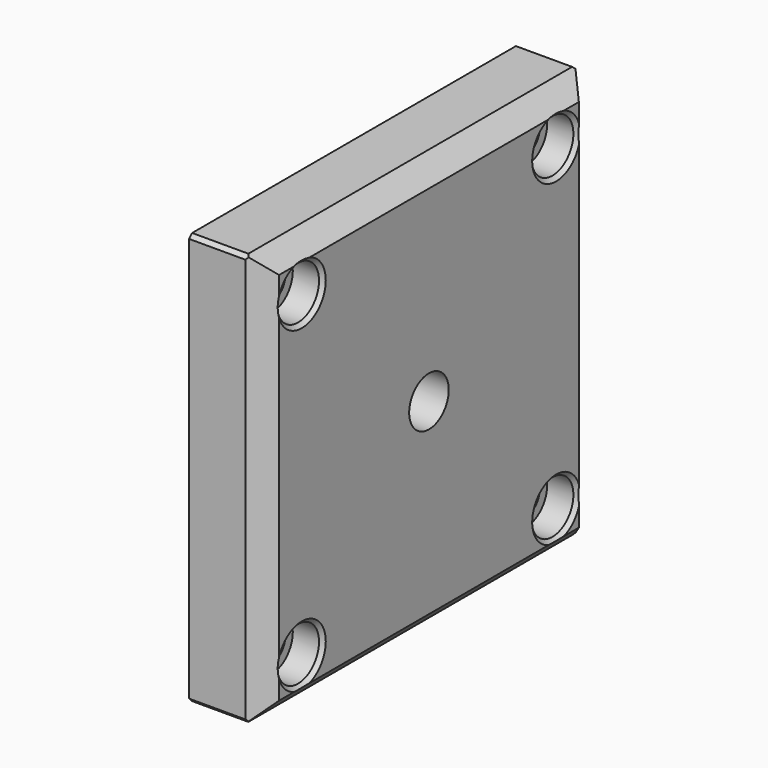
from build123d import *

# Parameters (mm, degrees)
F0_W        = 110
F0_H        = 110
F0_R        = 7
F0_R_2      = 6.6
F0_R_3      = 4.5
F0_R_4      = 5.5
F1_DEPTH    = 20
F2_DEPTH    = 20.001
F3_DEPTH    = 8
F4_DEPTH    = 9.4
F5_SIZE     = 1
F6_T1_DEPTH = 133.7168298797
F6_T3_DEPTH = 133.7168298797
F7_SIZE     = 0.5


# Not quite as in the source:
# - a fillet or chamfer that OpenCascade refuses, or shapes differently, is made with other operations: its cross-section is extruded or revolved along the edge and cut away or added


with BuildPart() as f1:
    # F0 (on Right) → F1 (new body)
    with BuildSketch(Plane.YZ):
        Rectangle(F0_W, F0_H)
        with Locations((-42.4264068712, -42.4264068712)):
            Circle(F0_R, mode=Mode.SUBTRACT)
        with Locations((42.4264068712, -42.4264068712)):
            Circle(F0_R, mode=Mode.SUBTRACT)
        with Locations((-42.4264068712, 42.4264068712)):
            Circle(F0_R, mode=Mode.SUBTRACT)
        Circle(F0_R_2, mode=Mode.SUBTRACT)
        with Locations((42.4264068712, 42.4264068712)):
            Circle(F0_R, mode=Mode.SUBTRACT)
        with Locations((-42.4264068712, 42.4264068712)):
            Circle(F0_R)
        with Locations((-42.4264068712, 42.4264068712)):
            Circle(F0_R_3, mode=Mode.SUBTRACT)
        with Locations((-42.4264068712, -42.4264068712)):
            Circle(F0_R)
        with Locations((-42.4264068712, -42.4264068712)):
            Circle(F0_R_3, mode=Mode.SUBTRACT)
        with Locations((42.4264068712, -42.4264068712)):
            Circle(F0_R)
        with Locations((42.4264068712, -42.4264068712)):
            Circle(F0_R_3, mode=Mode.SUBTRACT)
        with Locations((42.4264068712, 42.4264068712)):
            Circle(F0_R)
        with Locations((42.4264068712, 42.4264068712)):
            Circle(F0_R_3, mode=Mode.SUBTRACT)
        Circle(F0_R_2)
        Circle(F0_R_4, mode=Mode.SUBTRACT)
        Circle(F0_R_4)
        with Locations((-42.4264068712, 42.4264068712)):
            Circle(F0_R_3)
        with Locations((-42.4264068712, -42.4264068712)):
            Circle(F0_R_3)
        with Locations((42.4264068712, -42.4264068712)):
            Circle(F0_R_3)
        with Locations((42.4264068712, 42.4264068712)):
            Circle(F0_R_3)
    extrude(amount=-F1_DEPTH)

    # F0 (on Right) → F2 (cut, through all)
    with BuildSketch(Plane.YZ):
        with Locations((-42.4264068712, 42.4264068712)):
            Circle(F0_R_3)
        with Locations((42.4264068712, -42.4264068712)):
            Circle(F0_R_3)
        with Locations((-42.4264068712, -42.4264068712)):
            Circle(F0_R_3)
        Circle(F0_R_4)
        with Locations((42.4264068712, 42.4264068712)):
            Circle(F0_R_3)
    extrude(amount=-F2_DEPTH, mode=Mode.SUBTRACT)

    # F0 (on Right) → F3 (cut)
    with BuildSketch(Plane.YZ):
        with Locations((-42.4264068712, 42.4264068712)):
            Circle(F0_R)
        with Locations((-42.4264068712, 42.4264068712)):
            Circle(F0_R_3, mode=Mode.SUBTRACT)
        with Locations((42.4264068712, 42.4264068712)):
            Circle(F0_R)
        with Locations((42.4264068712, 42.4264068712)):
            Circle(F0_R_3, mode=Mode.SUBTRACT)
        with Locations((-42.4264068712, -42.4264068712)):
            Circle(F0_R)
        with Locations((-42.4264068712, -42.4264068712)):
            Circle(F0_R_3, mode=Mode.SUBTRACT)
        with Locations((42.4264068712, -42.4264068712)):
            Circle(F0_R)
        with Locations((42.4264068712, -42.4264068712)):
            Circle(F0_R_3, mode=Mode.SUBTRACT)
    extrude(amount=-F3_DEPTH, mode=Mode.SUBTRACT)

    # F0 (on Right) → F4 (cut)
    with BuildSketch(Plane.YZ):
        Circle(F0_R_2)
        Circle(F0_R_4, mode=Mode.SUBTRACT)
    extrude(amount=-F4_DEPTH, mode=Mode.SUBTRACT)

    # F5
    f5_edges = [f1.edges().sort_by_distance(p)[0] for p in [
        (0, -49.426407, 42.426407),
        (0, 35.426407, 42.426407),
        (0, -49.426407, -42.426407),
        (0, 35.426407, -42.426407),
        (-10, 55, -55),
        (-10, 55, 55),
        (-10, -55, 55),
        (-10, -55, -55),
    ]]
    chamfer(f5_edges, length=F5_SIZE)

    # F6: chamfer of 5 on 4 edges, made by hand

    # F6_s2 → F6_t1 (cut)
    with BuildSketch(Plane.XY.offset(-66.8584149398)):
        Polygon((0, -50), (-5, -55), (0, -55), align=None)
        Polygon((-5, 55), (0, 50), (0, 55), align=None)
    extrude(amount=F6_T1_DEPTH, mode=Mode.SUBTRACT)

    # F6_s4 → F6_t3 (cut)
    with BuildSketch(Plane.XZ.offset(-66.8584149398)):
        Polygon((0, 50), (-5, 55), (0, 55), align=None)
        Polygon((0, -50), (-5, -55), (0, -55), align=None)
    extrude(amount=F6_T3_DEPTH, mode=Mode.SUBTRACT)

    # F7
    f7_edges = [f1.edges().sort_by_distance(p)[0] for p in [
        (-20, 37.926407, -42.426407),
        (-20, 37.926407, 42.426407),
        (-20, -46.926407, 42.426407),
        (-20, -46.926407, -42.426407),
        (-20, -5.5, 0),
    ]]
    chamfer(f7_edges, length=F7_SIZE)


solid = f1.part
